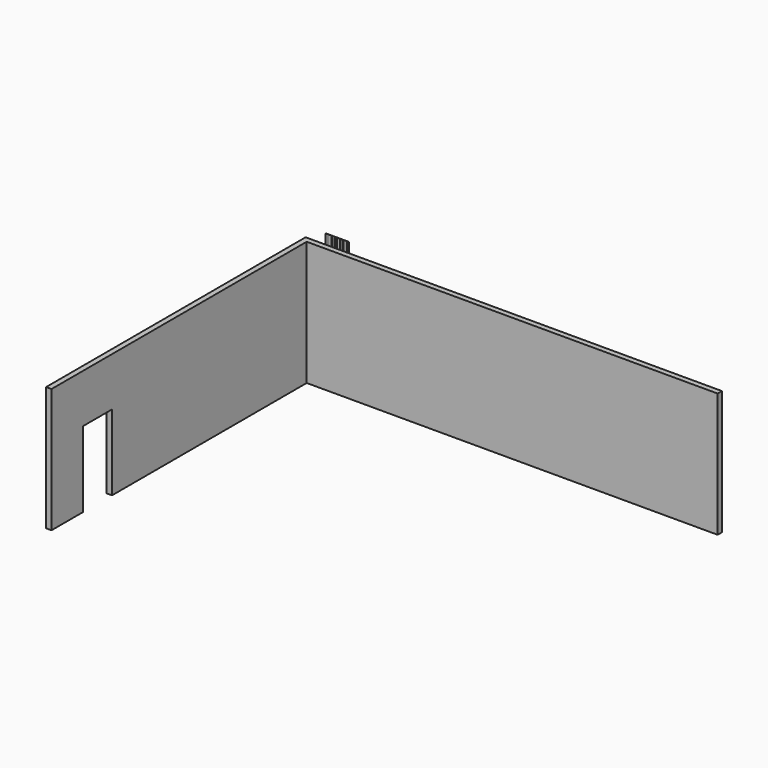
from build123d import *

# Parameters (mm, degrees)
F1_DEPTH    = 3505.2
F2_W        = 1016
F2_H        = 2133.6
F3_DEPTH    = 203.2
F5_DEPTH    = 3505.2
F6_T        = -4.7752
F7_R        = 3.175
F8_T1_DEPTH = 3495.6496


# Not quite as in the source:
# - a fillet or chamfer that OpenCascade refuses, or shapes differently, is made with other operations: its cross-section is extruded or revolved along the edge and cut away or added


with BuildPart() as f1:
    # F0 (on Top) → F1 (new body)
    with BuildSketch(Plane.XY):
        Polygon((0, 8991.6), (0, 0), (152.4, 0), (152.4, 8991.6), (11734.8, 8991.6), (11734.8, 9144), (152.4, 9144), (0, 9144), align=None)
    extrude(amount=F1_DEPTH)

    # F2 (on face) → F3 (cut)
    with BuildSketch(Plane(origin=(0, 0, 0), x_dir=(0, -1, 0), z_dir=(-1, 0, 0))):
        with Locations((-1625.6, 1066.8)):
            Rectangle(F2_W, F2_H)
    extrude(amount=-F3_DEPTH, mode=Mode.SUBTRACT)


with BuildPart() as f5:
    # F4 (on Top) → F5 (new body)
    with BuildSketch(Plane.XY):
        with BuildLine():
            Line((221.4464992285, 9568.2091308594), (221.4464992285, 9561.8591308594))
            Line((221.4464992285, 9561.8591308594), (291.2964992285, 9561.8591308594))
            Line((291.2964992285, 9561.8591308594), (296.7165632587, 9556.4390668291))
            ThreePointArc((296.7165632587, 9556.4390668291), (297.7466073913, 9555.7508133437), (298.961627289, 9555.5091308594))
            Line((298.961627289, 9555.5091308594), (309.0313711679, 9555.5091308594))
            ThreePointArc((309.0313711679, 9555.5091308594), (310.2463910657, 9555.7508133437), (311.2764351982, 9556.4390668291))
            Line((311.2764351982, 9556.4390668291), (316.6964992285, 9561.8591308594))
            Line((316.6964992285, 9561.8591308594), (380.1964992285, 9561.8591308594))
            Line((380.1964992285, 9561.8591308594), (385.6165632587, 9556.4390668291))
            ThreePointArc((385.6165632587, 9556.4390668291), (386.6466073913, 9555.7508133437), (387.861627289, 9555.5091308594))
            Line((387.861627289, 9555.5091308594), (397.9313711679, 9555.5091308594))
            ThreePointArc((397.9313711679, 9555.5091308594), (399.1463910657, 9555.7508133437), (400.1764351982, 9556.4390668291))
            Line((400.1764351982, 9556.4390668291), (405.5964992285, 9561.8591308594))
            Line((405.5964992285, 9561.8591308594), (475.4464992285, 9561.8591308594))
            Line((475.4464992285, 9561.8591308594), (499.9165632587, 9537.3890668291))
            ThreePointArc((499.9165632587, 9537.3890668291), (500.9466073913, 9536.7008133437), (502.161627289, 9536.4591308594))
            Line((502.161627289, 9536.4591308594), (524.9313711679, 9536.4591308594))
            ThreePointArc((524.9313711679, 9536.4591308594), (526.1463910657, 9536.7008133437), (527.1764351982, 9537.3890668291))
            Line((527.1764351982, 9537.3890668291), (551.6464992285, 9561.8591308594))
            Line((551.6464992285, 9561.8591308594), (621.4964992285, 9561.8591308594))
            Line((621.4964992285, 9561.8591308594), (626.9165632588, 9556.4390668291))
            ThreePointArc((626.9165632588, 9556.4390668291), (627.9466073913, 9555.7508133437), (629.161627289, 9555.5091308594))
            Line((629.161627289, 9555.5091308594), (639.2313711679, 9555.5091308594))
            ThreePointArc((639.2313711679, 9555.5091308594), (640.4463910657, 9555.7508133437), (641.4764351982, 9556.4390668291))
            Line((641.4764351982, 9556.4390668291), (646.8964992285, 9561.8591308594))
            Line((646.8964992285, 9561.8591308594), (710.3964992285, 9561.8591308594))
            Line((710.3964992285, 9561.8591308594), (714.886627289, 9557.3690027988))
            ThreePointArc((714.886627289, 9557.3690027988), (715.9166714215, 9556.6807493134), (717.1316913193, 9556.4390668291))
            Line((717.1316913193, 9556.4390668291), (724.5711790772, 9556.4390668291))
            ThreePointArc((724.5711790772, 9556.4390668291), (725.7861989749, 9556.6807493134), (726.8162431074, 9557.3690027988))
            Line((726.8162431074, 9557.3690027988), (731.306371168, 9561.8591308594))
            Line((731.306371168, 9561.8591308594), (805.6464992285, 9561.8591308594))
            Line((805.6464992285, 9561.8591308594), (829.186627289, 9538.3190027988))
            ThreePointArc((829.186627289, 9538.3190027988), (830.2166714215, 9537.6307493134), (831.4316913193, 9537.3890668291))
            Line((831.4316913193, 9537.3890668291), (851.5711790771, 9537.3890668291))
            ThreePointArc((851.5711790771, 9537.3890668291), (852.7861989749, 9537.6307493134), (853.8162431074, 9538.3190027988))
            Line((853.8162431074, 9538.3190027988), (877.3563711679, 9561.8591308594))
            Line((877.3563711679, 9561.8591308594), (877.3563711679, 9568.2091308594))
            Line((877.3563711679, 9568.2091308594), (221.4464992285, 9568.2091308594))
        make_face()
    extrude(amount=F5_DEPTH)

    # F6
    f6_openings = [f5.faces().sort_by_distance(p)[0] for p in [
        (549.401435, 9568.209131, 1752.6),
    ]]
    offset(amount=F6_T, openings=f6_openings, kind=Kind.INTERSECTION)

    # F7
    f7_edges = [f5.edges().sort_by_distance(p)[0] for p in [
        (805.646499, 9561.859131, 1752.6),
        (731.306371, 9561.859131, 1752.6),
        (710.396499, 9561.859131, 1752.6),
        (646.896499, 9561.859131, 1752.6),
        (621.496499, 9561.859131, 1752.6),
        (551.646499, 9561.859131, 1752.6),
        (475.446499, 9561.859131, 1752.6),
        (405.596499, 9561.859131, 1752.6),
        (380.196499, 9561.859131, 1752.6),
        (316.696499, 9561.859131, 1752.6),
        (291.296499, 9561.859131, 1752.6),
    ]]
    fillet(f7_edges, radius=F7_R)

    # F8: fillet of radius 5.08 on 12 edges, made by hand

    # F8_s2 → F8_t1 (cut)
    with BuildSketch(Plane.XY.offset(4.7752)):
        with BuildLine():
            ThreePointArc((294.7623493831, 9565.1464333078), (293.1142787711, 9566.2476388845), (291.1702469347, 9566.6343308594))
            Line((291.1702469347, 9566.6343308594), (293.2744518315, 9566.6343308594))
            Line((293.2744518315, 9566.6343308594), (294.7623493831, 9565.1464333078))
        make_face()
        with BuildLine():
            ThreePointArc((475.3202469347, 9566.6343308594), (477.2642787711, 9566.2476388845), (478.9123493831, 9565.1464333078))
            Line((478.9123493831, 9565.1464333078), (477.4244518315, 9566.6343308594))
            Line((477.4244518315, 9566.6343308594), (475.3202469347, 9566.6343308594))
        make_face()
        with BuildLine():
            ThreePointArc((548.1806490739, 9565.1464333078), (549.8287196859, 9566.2476388845), (551.7727515223, 9566.6343308594))
            Line((551.7727515223, 9566.6343308594), (549.6685466254, 9566.6343308594))
            Line((549.6685466254, 9566.6343308594), (548.1806490739, 9565.1464333078))
        make_face()
        with BuildLine():
            ThreePointArc((621.3702469347, 9566.6343308594), (623.3142787711, 9566.2476388845), (624.9623493831, 9565.1464333078))
            Line((624.9623493831, 9565.1464333078), (623.4744518315, 9566.6343308594))
            Line((623.4744518315, 9566.6343308594), (621.3702469347, 9566.6343308594))
        make_face()
        with BuildLine():
            ThreePointArc((710.2702469347, 9566.6343308594), (712.2142787711, 9566.2476388845), (713.8623493831, 9565.1464333078))
            Line((713.8623493831, 9565.1464333078), (712.3744518315, 9566.6343308594))
            Line((712.3744518315, 9566.6343308594), (710.2702469347, 9566.6343308594))
        make_face()
        with BuildLine():
            ThreePointArc((805.5202469347, 9566.6343308594), (807.4642787711, 9566.2476388845), (809.1123493831, 9565.1464333078))
            Line((809.1123493831, 9565.1464333078), (807.6244518315, 9566.6343308594))
            Line((807.6244518315, 9566.6343308594), (805.5202469347, 9566.6343308594))
        make_face()
        with BuildLine():
            ThreePointArc((877.6115988945, 9568.2091308594), (874.2791822956, 9566.9633712811), (872.5811711679, 9563.8370834624))
            Line((872.5811711679, 9563.8370834624), (872.5811711679, 9568.2091308594))
            Line((872.5811711679, 9568.2091308594), (877.6115988945, 9568.2091308594))
        make_face()
        with BuildLine():
            ThreePointArc((313.2306490739, 9565.1464333078), (314.8787196859, 9566.2476388845), (316.8227515223, 9566.6343308594))
            Line((316.8227515223, 9566.6343308594), (314.7185466254, 9566.6343308594))
            Line((314.7185466254, 9566.6343308594), (313.2306490739, 9565.1464333078))
        make_face()
        with BuildLine():
            ThreePointArc((380.0702469347, 9566.6343308594), (382.0142787711, 9566.2476388845), (383.6623493831, 9565.1464333078))
            Line((383.6623493831, 9565.1464333078), (382.1744518315, 9566.6343308594))
            Line((382.1744518315, 9566.6343308594), (380.0702469347, 9566.6343308594))
        make_face()
        with BuildLine():
            ThreePointArc((402.1306490739, 9565.1464333078), (403.7787196859, 9566.2476388845), (405.7227515223, 9566.6343308594))
            Line((405.7227515223, 9566.6343308594), (403.6185466254, 9566.6343308594))
            Line((403.6185466254, 9566.6343308594), (402.1306490739, 9565.1464333078))
        make_face()
        with BuildLine():
            ThreePointArc((643.4306490739, 9565.1464333078), (645.0787196859, 9566.2476388845), (647.0227515223, 9566.6343308594))
            Line((647.0227515223, 9566.6343308594), (644.9185466254, 9566.6343308594))
            Line((644.9185466254, 9566.6343308594), (643.4306490739, 9565.1464333078))
        make_face()
        with BuildLine():
            ThreePointArc((727.8405210133, 9565.1464333078), (729.4885916254, 9566.2476388845), (731.4326234618, 9566.6343308594))
            Line((731.4326234618, 9566.6343308594), (729.3284185649, 9566.6343308594))
            Line((729.3284185649, 9566.6343308594), (727.8405210133, 9565.1464333078))
        make_face()
    extrude(amount=F8_T1_DEPTH, mode=Mode.SUBTRACT)


solid = Compound([f1.part, f5.part])
